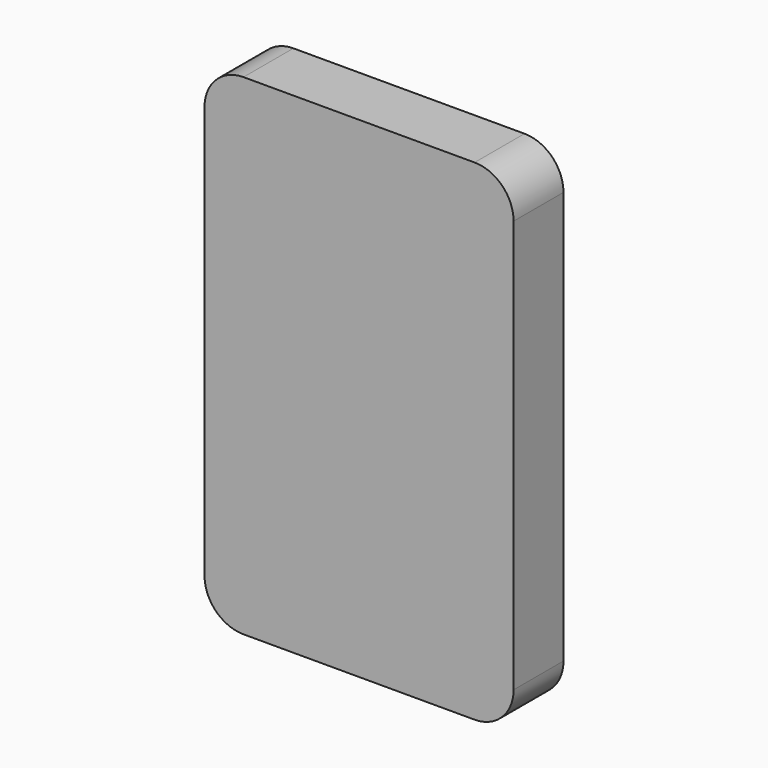
from build123d import *

# Parameters (mm, degrees)
F0_W     = 39.643229451
F0_H     = 62.91637104
F1_DEPTH = 3
F2_R     = 5
F3_R     = 1.2078964804
F3_R_2   = 1.1945278086
F3_R_3   = 1.7688403941
F3_R_4   = 5.8693557263
F3_R_5   = 3.6035226858
F3_R_6   = 3.4212098418
F5_DEPTH = 3
F6_DEPTH = 5


# Not quite as in the source:
# - the program builds the solid bodies; features that only make, move or delete a surface that nothing else refers to are left out


with BuildPart() as f1:
    # F0 (on Front) → F1 (new body)
    with BuildSketch(Plane.XZ):
        with Locations((-25.5412899423, 17.5534696318)):
            Rectangle(F0_W, F0_H)
    extrude(amount=F1_DEPTH)

    # F2
    f2_edges = [f1.edges().sort_by_distance(p)[0] for p in [
        (-45.362905, -1.5, 49.011655),
        (-45.362905, -1.5, -13.904716),
        (-5.719675, -1.5, -13.904716),
        (-5.719675, -1.5, 49.011655),
    ]]
    fillet(f2_edges, radius=F2_R)

    # F3 (on face) → F5 (join)
    with BuildSketch(Plane(origin=(0, 0, 0), x_dir=(-1, 0, 0), z_dir=(0, 1, 0))):
        with Locations((38.1972528994, 45.2637411654)):
            Circle(F3_R)
        with Locations((35.0141488016, 44.0116551518)):
            Circle(F3_R_2)
        with Locations((30.9397745878, 45.2637411654)):
            Circle(F3_R_3)
        with Locations((23.9369440824, 35.4597829282)):
            Circle(F3_R_4)
        with Locations((35.1414717734, 35.7144325972)):
            Circle(F3_R_5)
        with Locations((10.6952302158, 35.7144325972)):
            Circle(F3_R_6)
    extrude(amount=F5_DEPTH)

    # F6 (add): a face of the model
    f6_faces = [f1.faces().sort_by_distance(p)[0] for p in [
        (-25.6181685943, 0, 15.8495495724),
    ]]
    extrude(f6_faces, amount=F6_DEPTH)


solid = f1.part
